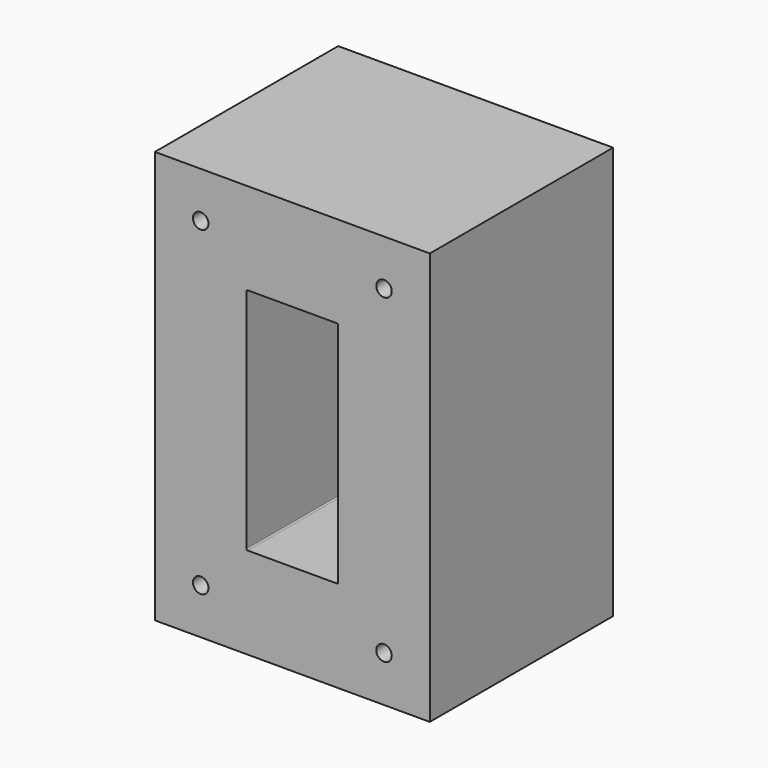
from build123d import *

# Parameters (mm, degrees)
F2_W     = 182.88
F2_H     = 274.32
F3_DEPTH = 152.4
F4_R     = 5.159375
F5_DEPTH = 152.4
F6_W     = 60.96
F6_H     = 152.4
F7_DEPTH = 152.4
F8_R     = 0.79375


with BuildPart() as f3:
    # F2 (on Front) → F3 (new body)
    with BuildSketch(Plane.XZ):
        Rectangle(F2_W, F2_H)
    extrude(amount=-F3_DEPTH)

    # F4 (on face) → F5 (cut)
    with BuildSketch(Plane.XZ):
        with Locations((-60.96, 106.68)):
            Circle(F4_R)
        with Locations((60.96, 106.68)):
            Circle(F4_R)
        with Locations((-60.96, -106.68)):
            Circle(F4_R)
        with Locations((60.96, -106.68)):
            Circle(F4_R)
    extrude(amount=-F5_DEPTH, mode=Mode.SUBTRACT)

    # F6 (on face) → F7 (cut)
    with BuildSketch(Plane.XZ):
        Rectangle(F6_W, F6_H)
    extrude(amount=-F7_DEPTH, mode=Mode.SUBTRACT)

    # F8
    f8_edges = [f3.edges().sort_by_distance(p)[0] for p in [
        (-30.48, 76.2, 76.2),
        (30.48, 76.2, 76.2),
        (30.48, 76.2, -76.2),
        (-30.48, 76.2, -76.2),
    ]]
    fillet(f8_edges, radius=F8_R)


solid = f3.part
